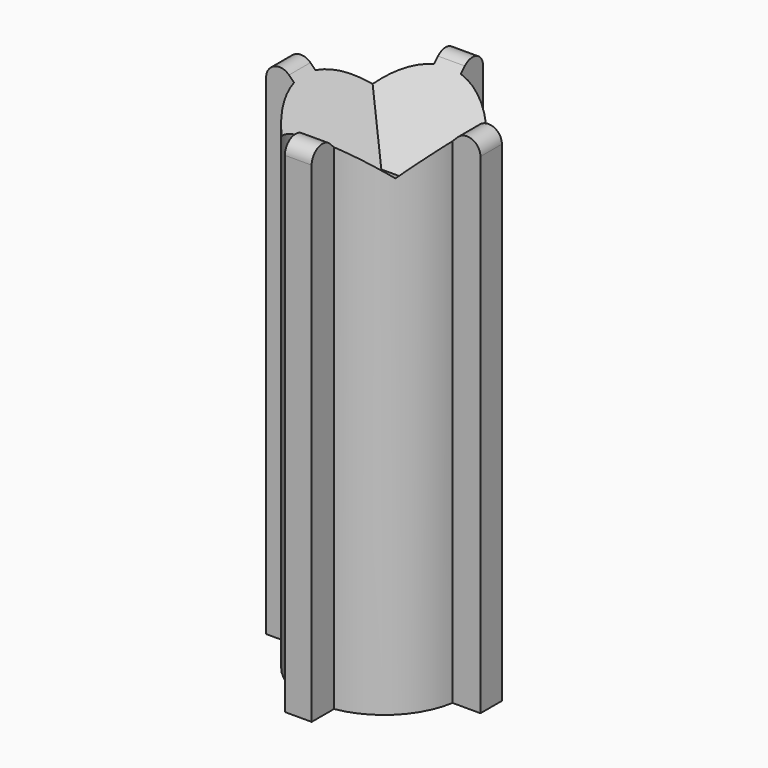
from build123d import *

# Parameters (mm, degrees)
F1_DEPTH     = 25.4
F2_T1_DEPTH  = 1.27
F2_T3_DEPTH  = 1.27
F2_T9_DEPTH  = 14.3341495789
F2_S10_R     = 3.81
F2_T11_DEPTH = 10
F2_T15_DEPTH = 14.3341495789
F2_S16_R     = 3.81
F2_T17_DEPTH = 10
F2_T24_DEPTH = 14.3341495789
F2_S25_R     = 3.81
F2_T26_DEPTH = 10
F2_T30_DEPTH = 14.3341495789
F2_S31_R     = 3.81
F2_T32_DEPTH = 10
F2_T39_DEPTH = 14.3341495789
F2_S40_R     = 3.81
F2_T41_DEPTH = 10
F2_T45_DEPTH = 14.3341495789
F2_S46_R     = 3.81
F2_T47_DEPTH = 10
F2_T54_DEPTH = 14.3341495789
F2_S55_R     = 3.81
F2_T56_DEPTH = 10
F2_T60_DEPTH = 14.3341495789
F2_S61_R     = 3.81
F2_T62_DEPTH = 10
F3_R         = 0.635


# Not quite as in the source:
# - a fillet or chamfer that OpenCascade refuses, or shapes differently, is made with other operations: its cross-section is extruded or revolved along the edge and cut away or added


with BuildPart() as f1:
    # F0 (on Top) → F1 (new body)
    with BuildSketch(Plane.XY):
        with BuildLine():
            ThreePointArc((3.7567106623, -0.635), (3.7966542918, -0.3186160517), (3.81, 0))
            ThreePointArc((3.81, 0), (3.7966542918, 0.3186160517), (3.7567106623, 0.635))
            Line((3.7567106623, 0.635), (0.635, 0.635))
            Line((0.635, 0.635), (0.635, -0.635))
            Line((0.635, -0.635), (3.7567106623, -0.635))
        make_face()
        with BuildLine():
            ThreePointArc((3.7567106623, 0.635), (3.7966542918, 0.3186160517), (3.81, 0))
            ThreePointArc((3.81, 0), (3.7966542918, -0.3186160517), (3.7567106623, -0.635))
            Line((3.7567106623, -0.635), (5.08, -0.635))
            Line((5.08, -0.635), (5.08, 0.635))
            Line((5.08, 0.635), (3.7567106623, 0.635))
        make_face()
        with BuildLine():
            Line((0.635, 0.635), (3.7567106623, 0.635))
            ThreePointArc((3.7567106623, 0.635), (2.6940768363, 2.6940768363), (0.635, 3.7567106623))
            Line((0.635, 3.7567106623), (0.635, 0.635))
        make_face()
        with BuildLine():
            ThreePointArc((0.635, -3.7567106623), (2.6940768363, -2.6940768363), (3.7567106623, -0.635))
            Line((3.7567106623, -0.635), (0.635, -0.635))
            Line((0.635, -0.635), (0.635, -3.7567106623))
        make_face()
        with BuildLine():
            Line((0.635, 0.635), (0.635, 3.7567106623))
            ThreePointArc((0.635, 3.7567106623), (0, 3.81), (-0.635, 3.7567106623))
            Line((-0.635, 3.7567106623), (-0.635, 0.635))
            Line((-0.635, 0.635), (0.635, 0.635))
        make_face()
        with BuildLine():
            ThreePointArc((-0.635, 3.7567106623), (0, 3.81), (0.635, 3.7567106623))
            Line((0.635, 3.7567106623), (0.635, 5.08))
            Line((0.635, 5.08), (-0.635, 5.08))
            Line((-0.635, 5.08), (-0.635, 3.7567106623))
        make_face()
        with BuildLine():
            Line((0.635, -5.08), (0.635, -3.7567106623))
            ThreePointArc((0.635, -3.7567106623), (0, -3.81), (-0.635, -3.7567106623))
            Line((-0.635, -3.7567106623), (-0.635, -5.08))
            Line((-0.635, -5.08), (0.635, -5.08))
        make_face()
        with BuildLine():
            ThreePointArc((-0.635, -3.7567106623), (0, -3.81), (0.635, -3.7567106623))
            Line((0.635, -3.7567106623), (0.635, -0.635))
            Line((0.635, -0.635), (-0.635, -0.635))
            Line((-0.635, -0.635), (-0.635, -3.7567106623))
        make_face()
        with BuildLine():
            Line((-0.635, 0.635), (-0.635, 3.7567106623))
            ThreePointArc((-0.635, 3.7567106623), (-2.6940768363, 2.6940768363), (-3.7567106623, 0.635))
            Line((-3.7567106623, 0.635), (-0.635, 0.635))
        make_face()
        with BuildLine():
            Line((-0.635, -0.635), (-0.635, 0.635))
            Line((-0.635, 0.635), (-3.7567106623, 0.635))
            ThreePointArc((-3.7567106623, 0.635), (-3.81, 0), (-3.7567106623, -0.635))
            Line((-3.7567106623, -0.635), (-0.635, -0.635))
        make_face()
        with BuildLine():
            ThreePointArc((-3.7567106623, -0.635), (-2.6940768363, -2.6940768363), (-0.635, -3.7567106623))
            Line((-0.635, -3.7567106623), (-0.635, -0.635))
            Line((-0.635, -0.635), (-3.7567106623, -0.635))
        make_face()
        with BuildLine():
            ThreePointArc((-3.7567106623, -0.635), (-3.81, 0), (-3.7567106623, 0.635))
            Line((-3.7567106623, 0.635), (-5.08, 0.635))
            Line((-5.08, 0.635), (-5.08, -0.635))
            Line((-5.08, -0.635), (-3.7567106623, -0.635))
        make_face()
    extrude(amount=F1_DEPTH)

    # F2: chamfer of 5.08 on 4 edges, made by hand

    # F2_s2 → F2_t1 (cut)
    with BuildSketch(Plane.YZ.offset(-0.635)):
        Polygon((0.635, 20.32), (5.715, 25.4), (0.635, 25.4), align=None)
        Polygon((-0.635, 20.32), (-5.715, 25.4), (-0.635, 25.4), align=None)
    extrude(amount=F2_T1_DEPTH, mode=Mode.SUBTRACT)

    # F2_s4 → F2_t3 (cut)
    with BuildSketch(Plane.XZ.offset(-0.635)):
        Polygon((-0.635, 20.32), (-5.715, 25.4), (-0.635, 25.4), align=None)
        Polygon((0.635, 20.32), (5.715, 25.4), (0.635, 25.4), align=None)
    extrude(amount=F2_T3_DEPTH, mode=Mode.SUBTRACT)


with BuildPart() as f2_tool7:
    # F2_s8 → F2_t9 (new body)
    with BuildSketch(Plane.XZ.offset(0.635)):
        Polygon((-0.635, 20.32), (-5.715, 25.4), (-0.635, 25.4), align=None)
    extrude(amount=-F2_T9_DEPTH)

    # F2_s10 → F2_t11 (intersect, symmetric)
    with BuildSketch(Plane.XY.offset(22.9)):
        Circle(F2_S10_R)
    extrude(amount=F2_T11_DEPTH, both=True, mode=Mode.INTERSECT)

    split(bisect_by=Plane.XZ.offset(-0.635), keep=Keep.BOTTOM)


with BuildPart() as f2_tool13:
    # F2_s14 → F2_t15 (new body)
    with BuildSketch(Plane.YZ.offset(-13.6991495789)):
        Polygon((0.635, 20.32), (5.715, 25.4), (0.635, 25.4), align=None)
    extrude(amount=F2_T15_DEPTH)

    # F2_s16 → F2_t17 (intersect, symmetric)
    with BuildSketch(Plane.XY.offset(22.9)):
        Circle(F2_S16_R)
    extrude(amount=F2_T17_DEPTH, both=True, mode=Mode.INTERSECT)

    split(bisect_by=Plane.YZ.offset(-0.635), keep=Keep.BOTTOM)


with BuildPart() as f2_tool7_1:
    add(f2_tool7.part)

    # F2_t19: intersect F2_tool13
    add(f2_tool13.part, mode=Mode.INTERSECT)


with BuildPart() as f1_1:
    add(f1.part)

    # F2_t5: cut F2_tool7
    add(f2_tool7_1.part, mode=Mode.SUBTRACT)


with BuildPart() as f2_tool22:
    # F2_s23 → F2_t24 (new body)
    with BuildSketch(Plane.YZ.offset(-0.635)):
        Polygon((0.635, 20.32), (5.715, 25.4), (0.635, 25.4), align=None)
    extrude(amount=F2_T24_DEPTH)

    # F2_s25 → F2_t26 (intersect, symmetric)
    with BuildSketch(Plane.XY.offset(22.9)):
        Circle(F2_S25_R)
    extrude(amount=F2_T26_DEPTH, both=True, mode=Mode.INTERSECT)

    split(bisect_by=Plane.YZ.offset(0.635), keep=Keep.TOP)


with BuildPart() as f2_tool28:
    # F2_s29 → F2_t30 (new body)
    with BuildSketch(Plane.XZ.offset(-13.6991495789)):
        Polygon((0.635, 20.32), (5.715, 25.4), (0.635, 25.4), align=None)
    extrude(amount=F2_T30_DEPTH)

    # F2_s31 → F2_t32 (intersect, symmetric)
    with BuildSketch(Plane.XY.offset(22.9)):
        Circle(F2_S31_R)
    extrude(amount=F2_T32_DEPTH, both=True, mode=Mode.INTERSECT)

    split(bisect_by=Plane.XZ.offset(-0.635), keep=Keep.BOTTOM)


with BuildPart() as f2_tool22_1:
    add(f2_tool22.part)

    # F2_t34: intersect F2_tool28
    add(f2_tool28.part, mode=Mode.INTERSECT)


with BuildPart() as f1_2:
    add(f1_1.part)

    # F2_t20: cut F2_tool22
    add(f2_tool22_1.part, mode=Mode.SUBTRACT)


with BuildPart() as f2_tool37:
    # F2_s38 → F2_t39 (new body)
    with BuildSketch(Plane.YZ.offset(0.635)):
        Polygon((-0.635, 20.32), (-5.715, 25.4), (-0.635, 25.4), align=None)
    extrude(amount=-F2_T39_DEPTH)

    # F2_s40 → F2_t41 (intersect, symmetric)
    with BuildSketch(Plane.XY.offset(22.9)):
        Circle(F2_S40_R)
    extrude(amount=F2_T41_DEPTH, both=True, mode=Mode.INTERSECT)

    split(bisect_by=Plane.YZ.offset(-0.635), keep=Keep.BOTTOM)


with BuildPart() as f2_tool43:
    # F2_s44 → F2_t45 (new body)
    with BuildSketch(Plane.XZ.offset(13.6991495789)):
        Polygon((-0.635, 20.32), (-5.715, 25.4), (-0.635, 25.4), align=None)
    extrude(amount=-F2_T45_DEPTH)

    # F2_s46 → F2_t47 (intersect, symmetric)
    with BuildSketch(Plane.XY.offset(22.9)):
        Circle(F2_S46_R)
    extrude(amount=F2_T47_DEPTH, both=True, mode=Mode.INTERSECT)

    split(bisect_by=Plane.XZ.offset(0.635), keep=Keep.TOP)


with BuildPart() as f2_tool37_1:
    add(f2_tool37.part)

    # F2_t49: intersect F2_tool43
    add(f2_tool43.part, mode=Mode.INTERSECT)


with BuildPart() as f1_3:
    add(f1_2.part)

    # F2_t35: cut F2_tool37
    add(f2_tool37_1.part, mode=Mode.SUBTRACT)


with BuildPart() as f2_tool52:
    # F2_s53 → F2_t54 (new body)
    with BuildSketch(Plane.YZ.offset(13.6991495789)):
        Polygon((-0.635, 20.32), (-5.715, 25.4), (-0.635, 25.4), align=None)
    extrude(amount=-F2_T54_DEPTH)

    # F2_s55 → F2_t56 (intersect, symmetric)
    with BuildSketch(Plane.XY.offset(22.9)):
        Circle(F2_S55_R)
    extrude(amount=F2_T56_DEPTH, both=True, mode=Mode.INTERSECT)

    split(bisect_by=Plane.YZ.offset(0.635), keep=Keep.TOP)


with BuildPart() as f2_tool58:
    # F2_s59 → F2_t60 (new body)
    with BuildSketch(Plane.XZ.offset(-0.635)):
        Polygon((0.635, 20.32), (5.715, 25.4), (0.635, 25.4), align=None)
    extrude(amount=F2_T60_DEPTH)

    # F2_s61 → F2_t62 (intersect, symmetric)
    with BuildSketch(Plane.XY.offset(22.9)):
        Circle(F2_S61_R)
    extrude(amount=F2_T62_DEPTH, both=True, mode=Mode.INTERSECT)

    split(bisect_by=Plane.XZ.offset(0.635), keep=Keep.TOP)


with BuildPart() as f2_tool52_1:
    add(f2_tool52.part)

    # F2_t64: intersect F2_tool58
    add(f2_tool58.part, mode=Mode.INTERSECT)


with BuildPart() as f1_4:
    add(f1_3.part)

    # F2_t50: cut F2_tool52
    add(f2_tool52_1.part, mode=Mode.SUBTRACT)

    # F3
    f3_edges = [f1_4.edges().sort_by_distance(p)[0] for p in [
        (5.08, 0, 24.765),
        (0, 5.08, 24.765),
        (-5.08, 0, 24.765),
        (0, -5.08, 24.765),
    ]]
    fillet(f3_edges, radius=F3_R)


solid = f1_4.part
